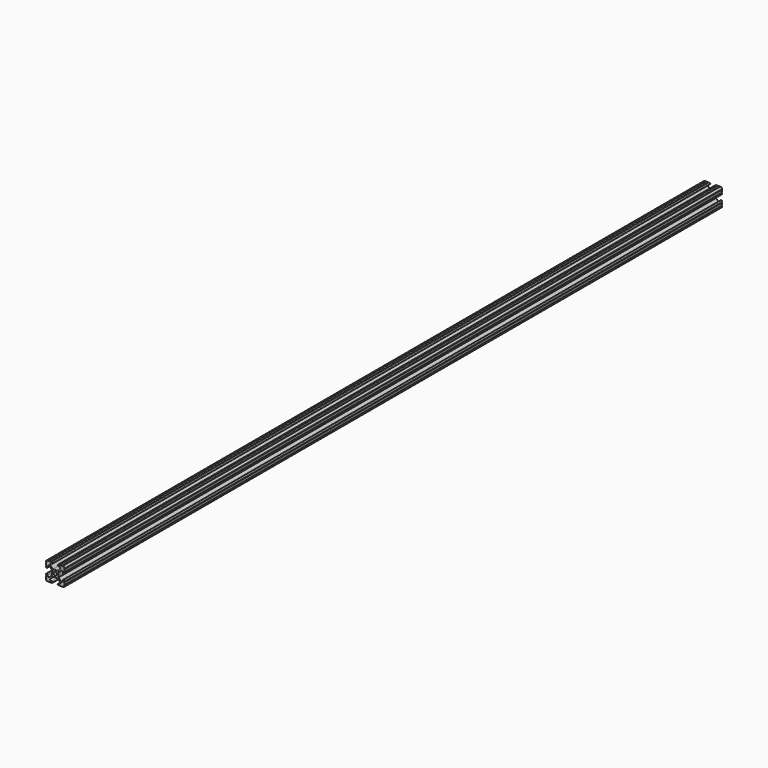
from build123d import *

# Parameters (mm, degrees)
F1_DEPTH    = 1143
F2_T1_DEPTH = 1143
F2_T3_DEPTH = 1150.9375
F2_T5_DEPTH = 1146.96875


# Not quite as in the source:
# - a fillet or chamfer that OpenCascade refuses, or shapes differently, is made with other operations: its cross-section is extruded or revolved along the edge and cut away or added


with BuildPart() as f1:
    # F0 (on Front) → F1 (new body)
    with BuildSketch(Plane.XZ):
        with BuildLine():
            ThreePointArc((-0.8361427067, 2.2296225996), (0, 2.38125), (0.8361427067, 2.2296225996))
            Line((0.8361427067, 2.2296225996), (3.1853789104, 4.5640625))
            Line((3.1853789104, 4.5640625), (-3.1853789104, 4.5640625))
            Line((-3.1853789104, 4.5640625), (-0.8361427067, 2.2296225996))
        make_face()
        with BuildLine():
            ThreePointArc((-2.2347427098, 0.8223603732), (-1.6889881746, 1.6785918231), (-0.8361427067, 2.2296225996))
            Line((-0.8361427067, 2.2296225996), (-3.1853789104, 4.5640625))
            Line((-3.1853789104, 4.5640625), (-4.5640625, 4.5640625))
            Line((-4.5640625, 4.5640625), (-4.5640625, 3.1376763557))
            Line((-4.5640625, 3.1376763557), (-2.2347427098, 0.8223603732))
        make_face()
        with BuildLine():
            ThreePointArc((-2.2347427098, -0.8223603732), (-2.38125, 0), (-2.2347427098, 0.8223603732))
            Line((-2.2347427098, 0.8223603732), (-4.5640625, 3.1376763557))
            Line((-4.5640625, 3.1376763557), (-4.5640625, -3.1376763557))
            Line((-4.5640625, -3.1376763557), (-2.2347427098, -0.8223603732))
        make_face()
        with BuildLine():
            Line((-3.1853789104, -4.5640625), (-0.8361427067, -2.2296225996))
            ThreePointArc((-0.8361427067, -2.2296225996), (-1.6889881746, -1.6785918231), (-2.2347427098, -0.8223603732))
            Line((-2.2347427098, -0.8223603732), (-4.5640625, -3.1376763557))
            Line((-4.5640625, -3.1376763557), (-4.5640625, -4.5640625))
            Line((-4.5640625, -4.5640625), (-3.1853789104, -4.5640625))
        make_face()
        with BuildLine():
            Line((3.1853789104, -4.5640625), (0.8361427067, -2.2296225996))
            ThreePointArc((0.8361427067, -2.2296225996), (0, -2.38125), (-0.8361427067, -2.2296225996))
            Line((-0.8361427067, -2.2296225996), (-3.1853789104, -4.5640625))
            Line((-3.1853789104, -4.5640625), (3.1853789104, -4.5640625))
        make_face()
        with BuildLine():
            Line((4.5640625, -3.1376763557), (2.2347427098, -0.8223603732))
            ThreePointArc((2.2347427098, -0.8223603732), (1.6889881746, -1.6785918231), (0.8361427067, -2.2296225996))
            Line((0.8361427067, -2.2296225996), (3.1853789104, -4.5640625))
            Line((3.1853789104, -4.5640625), (4.5640625, -4.5640625))
            Line((4.5640625, -4.5640625), (4.5640625, -3.1376763557))
        make_face()
        with BuildLine():
            ThreePointArc((2.2347427098, 0.8223603732), (2.3443370748, 0.4176544533), (2.38125, 0))
            ThreePointArc((2.38125, 0), (2.3443370748, -0.4176544533), (2.2347427098, -0.8223603732))
            Line((2.2347427098, -0.8223603732), (4.5640625, -3.1376763557))
            Line((4.5640625, -3.1376763557), (4.5640625, 3.1376763557))
            Line((4.5640625, 3.1376763557), (2.2347427098, 0.8223603732))
        make_face()
        with BuildLine():
            ThreePointArc((0.8361427067, 2.2296225996), (1.6889881746, 1.6785918231), (2.2347427098, 0.8223603732))
            Line((2.2347427098, 0.8223603732), (4.5640625, 3.1376763557))
            Line((4.5640625, 3.1376763557), (4.5640625, 4.5640625))
            Line((4.5640625, 4.5640625), (3.1853789104, 4.5640625))
            Line((3.1853789104, 4.5640625), (0.8361427067, 2.2296225996))
        make_face()
        Polygon((4.5640625, 4.5640625), (4.5640625, 3.1376763557), (10.715625, 9.2522558281), (12.7, 11.2247008192), (12.7, 12.7), (11.3728841543, 12.7), (9.3759316558, 10.715625), (3.1853789104, 4.5640625), align=None)
        with BuildLine():
            Line((12.7, 11.2247008192), (10.715625, 9.2522558281))
            Line((10.715625, 9.2522558281), (10.715625, 7.14375))
            Line((10.715625, 7.14375), (10.715625, 3.175))
            Line((10.715625, 3.175), (12.7, 3.175))
            Line((12.7, 3.175), (12.7, 5.55625))
            ThreePointArc((12.7, 5.55625), (12.303125, 5.953125), (12.7, 6.35))
            Line((12.7, 6.35), (12.7, 9.525))
            ThreePointArc((12.7, 9.525), (12.303125, 9.921875), (12.7, 10.31875))
            Line((12.7, 10.31875), (12.7, 11.2247008192))
        make_face()
        with BuildLine():
            Line((7.14375, 10.715625), (9.3759316558, 10.715625))
            Line((9.3759316558, 10.715625), (11.3728841543, 12.7))
            Line((11.3728841543, 12.7), (10.31875, 12.7))
            ThreePointArc((10.31875, 12.7), (9.921875, 12.303125), (9.525, 12.7))
            Line((9.525, 12.7), (6.35, 12.7))
            ThreePointArc((6.35, 12.7), (5.953125, 12.303125), (5.55625, 12.7))
            Line((5.55625, 12.7), (3.175, 12.7))
            Line((3.175, 12.7), (3.175, 10.715625))
            Line((3.175, 10.715625), (7.14375, 10.715625))
        make_face()
        with BuildLine():
            Line((-11.3728841543, 12.7), (-9.3759316558, 10.715625))
            Line((-9.3759316558, 10.715625), (-7.14375, 10.715625))
            Line((-7.14375, 10.715625), (-3.175, 10.715625))
            Line((-3.175, 10.715625), (-3.175, 12.7))
            Line((-3.175, 12.7), (-5.55625, 12.7))
            ThreePointArc((-5.55625, 12.7), (-5.953125, 12.303125), (-6.35, 12.7))
            Line((-6.35, 12.7), (-7.14375, 12.7))
            Line((-7.14375, 12.7), (-9.525, 12.7))
            ThreePointArc((-9.525, 12.7), (-9.921875, 12.303125), (-10.31875, 12.7))
            Line((-10.31875, 12.7), (-11.3728841543, 12.7))
        make_face()
        Polygon((-4.5640625, 4.5640625), (-3.1853789104, 4.5640625), (-9.3759316558, 10.715625), (-11.3728841543, 12.7), (-12.7, 11.2247008192), (-10.715625, 9.2522558281), (-4.5640625, 3.1376763557), align=None)
        Polygon((-12.7, 11.2247008192), (-11.3728841543, 12.7), (-12.7, 12.7), align=None)
        with BuildLine():
            Line((-10.715625, 7.14375), (-10.715625, 9.2522558281))
            Line((-10.715625, 9.2522558281), (-12.7, 11.2247008192))
            Line((-12.7, 11.2247008192), (-12.7, 10.31875))
            ThreePointArc((-12.7, 10.31875), (-12.303125, 9.921875), (-12.7, 9.525))
            Line((-12.7, 9.525), (-12.7, 6.35))
            ThreePointArc((-12.7, 6.35), (-12.303125, 5.953125), (-12.7, 5.55625))
            Line((-12.7, 5.55625), (-12.7, 3.175))
            Line((-12.7, 3.175), (-10.715625, 3.175))
            Line((-10.715625, 3.175), (-10.715625, 7.14375))
        make_face()
        with BuildLine():
            Line((-12.7, -11.2247008192), (-10.715625, -9.2522558281))
            Line((-10.715625, -9.2522558281), (-10.715625, -7.14375))
            Line((-10.715625, -7.14375), (-10.715625, -3.175))
            Line((-10.715625, -3.175), (-12.7, -3.175))
            Line((-12.7, -3.175), (-12.7, -5.55625))
            ThreePointArc((-12.7, -5.55625), (-12.303125, -5.953125), (-12.7, -6.35))
            Line((-12.7, -6.35), (-12.7, -9.525))
            ThreePointArc((-12.7, -9.525), (-12.303125, -9.921875), (-12.7, -10.31875))
            Line((-12.7, -10.31875), (-12.7, -11.2247008192))
        make_face()
        Polygon((-9.3759316558, -10.715625), (-3.1853789104, -4.5640625), (-4.5640625, -4.5640625), (-4.5640625, -3.1376763557), (-10.715625, -9.2522558281), (-12.7, -11.2247008192), (-12.7, -12.7), (-11.3728841543, -12.7), align=None)
        with BuildLine():
            Line((-7.14375, -10.715625), (-9.3759316558, -10.715625))
            Line((-9.3759316558, -10.715625), (-11.3728841543, -12.7))
            Line((-11.3728841543, -12.7), (-10.31875, -12.7))
            ThreePointArc((-10.31875, -12.7), (-9.921875, -12.303125), (-9.525, -12.7))
            Line((-9.525, -12.7), (-6.35, -12.7))
            ThreePointArc((-6.35, -12.7), (-5.953125, -12.303125), (-5.55625, -12.7))
            Line((-5.55625, -12.7), (-3.175, -12.7))
            Line((-3.175, -12.7), (-3.175, -10.715625))
            Line((-3.175, -10.715625), (-7.14375, -10.715625))
        make_face()
        with BuildLine():
            Line((11.3728841543, -12.7), (9.3759316558, -10.715625))
            Line((9.3759316558, -10.715625), (7.14375, -10.715625))
            Line((7.14375, -10.715625), (3.175, -10.715625))
            Line((3.175, -10.715625), (3.175, -12.7))
            Line((3.175, -12.7), (5.55625, -12.7))
            ThreePointArc((5.55625, -12.7), (5.953125, -12.303125), (6.35, -12.7))
            Line((6.35, -12.7), (9.525, -12.7))
            ThreePointArc((9.525, -12.7), (9.921875, -12.303125), (10.31875, -12.7))
            Line((10.31875, -12.7), (11.3728841543, -12.7))
        make_face()
        Polygon((10.715625, -9.2522558281), (4.5640625, -3.1376763557), (4.5640625, -4.5640625), (3.1853789104, -4.5640625), (9.3759316558, -10.715625), (11.3728841543, -12.7), (12.7, -12.7), (12.7, -11.2247008192), align=None)
        with BuildLine():
            Line((10.715625, -7.14375), (10.715625, -9.2522558281))
            Line((10.715625, -9.2522558281), (12.7, -11.2247008192))
            Line((12.7, -11.2247008192), (12.7, -10.31875))
            ThreePointArc((12.7, -10.31875), (12.303125, -9.921875), (12.7, -9.525))
            Line((12.7, -9.525), (12.7, -6.35))
            ThreePointArc((12.7, -6.35), (12.303125, -5.953125), (12.7, -5.55625))
            Line((12.7, -5.55625), (12.7, -3.175))
            Line((12.7, -3.175), (10.715625, -3.175))
            Line((10.715625, -3.175), (10.715625, -7.14375))
        make_face()
    extrude(amount=F1_DEPTH)

    # F2: fillet of radius 1.5875 on 31 edges, made by hand

    # F2_s2 → F2_t1 (join)
    with BuildSketch(Plane.XZ):
        with BuildLine():
            ThreePointArc((-6.6451596968, 8.0020523886), (-6.9937960043, 9.7333175229), (-5.5261794807, 10.715625))
            Line((-5.5261794807, 10.715625), (-9.3759316558, 10.715625))
            Line((-9.3759316558, 10.715625), (-6.6451596968, 8.0020523886))
        make_face()
        with BuildLine():
            ThreePointArc((-8.0089825615, 6.5618856508), (-9.7378452755, 6.9017155215), (-10.715625, 5.4359742634))
            Line((-10.715625, 5.4359742634), (-10.715625, 9.2522558281))
            Line((-10.715625, 9.2522558281), (-8.0089825615, 6.5618856508))
        make_face()
        with BuildLine():
            ThreePointArc((5.5261794807, 10.715625), (6.9937960043, 9.7333175229), (6.6451596968, 8.0020523886))
            Line((6.6451596968, 8.0020523886), (9.3759316558, 10.715625))
            Line((9.3759316558, 10.715625), (5.5261794807, 10.715625))
        make_face()
        with BuildLine():
            ThreePointArc((8.0089825615, 6.5618856508), (9.7378452755, 6.9017155215), (10.715625, 5.4359742634))
            Line((10.715625, 5.4359742634), (10.715625, 9.2522558281))
            Line((10.715625, 9.2522558281), (8.0089825615, 6.5618856508))
        make_face()
        with BuildLine():
            ThreePointArc((10.715625, -5.4359742634), (9.7378452755, -6.9017155215), (8.0089825615, -6.5618856508))
            Line((8.0089825615, -6.5618856508), (10.715625, -9.2522558281))
            Line((10.715625, -9.2522558281), (10.715625, -5.4359742634))
        make_face()
        with BuildLine():
            ThreePointArc((6.6451596968, -8.0020523886), (6.9937960043, -9.7333175229), (5.5261794807, -10.715625))
            Line((5.5261794807, -10.715625), (9.3759316558, -10.715625))
            Line((9.3759316558, -10.715625), (6.6451596968, -8.0020523886))
        make_face()
        with BuildLine():
            ThreePointArc((-5.5261794807, -10.715625), (-6.9937960043, -9.7333175229), (-6.6451596968, -8.0020523886))
            Line((-6.6451596968, -8.0020523886), (-9.3759316558, -10.715625))
            Line((-9.3759316558, -10.715625), (-5.5261794807, -10.715625))
        make_face()
        with BuildLine():
            ThreePointArc((-8.0089825615, -6.5618856508), (-9.7378452755, -6.9017155215), (-10.715625, -5.4359742634))
            Line((-10.715625, -5.4359742634), (-10.715625, -9.2522558281))
            Line((-10.715625, -9.2522558281), (-8.0089825615, -6.5618856508))
        make_face()
        with BuildLine():
            ThreePointArc((-2.530750733, 4.5640625), (-3.1359432558, 4.6839459764), (-3.649730949, 5.0254898886))
            Line((-3.649730949, 5.0254898886), (-3.1853789104, 4.5640625))
            Line((-3.1853789104, 4.5640625), (-2.530750733, 4.5640625))
        make_face()
    extrude(amount=F2_T1_DEPTH)

    # F2_s4 → F2_t3 (cut)
    with BuildSketch(Plane.XZ.offset(-3.96875)):
        with BuildLine():
            ThreePointArc((-12.7, -11.1125), (-12.2350320151, -12.2350320151), (-11.1125, -12.7))
            Line((-11.1125, -12.7), (-12.7, -12.7))
            Line((-12.7, -12.7), (-12.7, -11.1125))
        make_face()
        with BuildLine():
            ThreePointArc((11.1125, -12.7), (12.2350320151, -12.2350320151), (12.7, -11.1125))
            Line((12.7, -11.1125), (12.7, -12.7))
            Line((12.7, -12.7), (11.1125, -12.7))
        make_face()
        with BuildLine():
            ThreePointArc((12.7, 11.1125), (12.2350320151, 12.2350320151), (11.1125, 12.7))
            Line((11.1125, 12.7), (12.7, 12.7))
            Line((12.7, 12.7), (12.7, 11.1125))
        make_face()
        with BuildLine():
            ThreePointArc((-12.7, 4.7625), (-12.2350320151, 3.6399679849), (-11.1125, 3.175))
            Line((-11.1125, 3.175), (-12.7, 3.175))
            Line((-12.7, 3.175), (-12.7, 4.7625))
        make_face()
        with BuildLine():
            ThreePointArc((-11.1125, -3.175), (-12.2350320151, -3.6399679849), (-12.7, -4.7625))
            Line((-12.7, -4.7625), (-12.7, -3.175))
            Line((-12.7, -3.175), (-11.1125, -3.175))
        make_face()
        with BuildLine():
            ThreePointArc((-12.303125, 3.175), (-11.1805929849, 3.6399679849), (-10.715625, 4.7625))
            Line((-10.715625, 4.7625), (-10.715625, 3.175))
            Line((-10.715625, 3.175), (-12.303125, 3.175))
        make_face()
        with BuildLine():
            ThreePointArc((-10.715625, -4.7625), (-11.1805929849, -3.6399679849), (-12.303125, -3.175))
            Line((-12.303125, -3.175), (-10.715625, -3.175))
            Line((-10.715625, -3.175), (-10.715625, -4.7625))
        make_face()
        with BuildLine():
            ThreePointArc((-3.175, -12.303125), (-3.6399679849, -11.1805929849), (-4.7625, -10.715625))
            Line((-4.7625, -10.715625), (-3.175, -10.715625))
            Line((-3.175, -10.715625), (-3.175, -12.303125))
        make_face()
        with BuildLine():
            ThreePointArc((-4.7625, -12.7), (-3.6399679849, -12.2350320151), (-3.175, -11.1125))
            Line((-3.175, -11.1125), (-3.175, -12.7))
            Line((-3.175, -12.7), (-4.7625, -12.7))
        make_face()
        with BuildLine():
            ThreePointArc((3.175, -11.1125), (3.6399679849, -12.2350320151), (4.7625, -12.7))
            Line((4.7625, -12.7), (3.175, -12.7))
            Line((3.175, -12.7), (3.175, -11.1125))
        make_face()
        with BuildLine():
            ThreePointArc((4.7625, -10.715625), (3.6399679849, -11.1805929849), (3.175, -12.303125))
            Line((3.175, -12.303125), (3.175, -10.715625))
            Line((3.175, -10.715625), (4.7625, -10.715625))
        make_face()
        with BuildLine():
            ThreePointArc((12.7, -4.7625), (12.2350320151, -3.6399679849), (11.1125, -3.175))
            Line((11.1125, -3.175), (12.7, -3.175))
            Line((12.7, -3.175), (12.7, -4.7625))
        make_face()
        with BuildLine():
            ThreePointArc((11.1125, 3.175), (12.2350320151, 3.6399679849), (12.7, 4.7625))
            Line((12.7, 4.7625), (12.7, 3.175))
            Line((12.7, 3.175), (11.1125, 3.175))
        make_face()
        with BuildLine():
            ThreePointArc((12.303125, -3.175), (11.1805929849, -3.6399679849), (10.715625, -4.7625))
            Line((10.715625, -4.7625), (10.715625, -3.175))
            Line((10.715625, -3.175), (12.303125, -3.175))
        make_face()
        with BuildLine():
            ThreePointArc((10.715625, 4.7625), (11.1805929849, 3.6399679849), (12.303125, 3.175))
            Line((12.303125, 3.175), (10.715625, 3.175))
            Line((10.715625, 3.175), (10.715625, 4.7625))
        make_face()
        with BuildLine():
            ThreePointArc((-4.7625, 10.715625), (-3.6399679849, 11.1805929849), (-3.175, 12.303125))
            Line((-3.175, 12.303125), (-3.175, 10.715625))
            Line((-3.175, 10.715625), (-4.7625, 10.715625))
        make_face()
        with BuildLine():
            ThreePointArc((-3.175, 11.1125), (-3.6399679849, 12.2350320151), (-4.7625, 12.7))
            Line((-4.7625, 12.7), (-3.175, 12.7))
            Line((-3.175, 12.7), (-3.175, 11.1125))
        make_face()
        with BuildLine():
            ThreePointArc((4.7625, 12.7), (3.6399679849, 12.2350320151), (3.175, 11.1125))
            Line((3.175, 11.1125), (3.175, 12.7))
            Line((3.175, 12.7), (4.7625, 12.7))
        make_face()
        with BuildLine():
            ThreePointArc((3.175, 12.303125), (3.6399679849, 11.1805929849), (4.7625, 10.715625))
            Line((4.7625, 10.715625), (3.175, 10.715625))
            Line((3.175, 10.715625), (3.175, 12.303125))
        make_face()
        with BuildLine():
            ThreePointArc((-11.1125, 12.7), (-12.2350320151, 12.2350320151), (-12.7, 11.1125))
            Line((-12.7, 11.1125), (-12.7, 12.7))
            Line((-12.7, 12.7), (-11.1125, 12.7))
        make_face()
    extrude(amount=F2_T3_DEPTH, mode=Mode.SUBTRACT)

    # F2_s6 → F2_t5 (cut)
    with BuildSketch(Plane.XZ.offset(-1.984375)):
        with BuildLine():
            ThreePointArc((-8.73125, 12.7), (-9.2332615786, 12.6185347357), (-9.68375, 12.3825))
            ThreePointArc((-9.68375, 12.3825), (-9.5668992086, 12.5225121043), (-9.525, 12.7))
            Line((-9.525, 12.7), (-8.73125, 12.7))
        make_face()
        with BuildLine():
            ThreePointArc((-10.16, 12.3825), (-10.6104884214, 12.6185347357), (-11.1125, 12.7))
            Line((-11.1125, 12.7), (-10.31875, 12.7))
            ThreePointArc((-10.31875, 12.7), (-10.2768507914, 12.5225121043), (-10.16, 12.3825))
        make_face()
    extrude(amount=F2_T5_DEPTH, mode=Mode.SUBTRACT)


solid = f1.part
